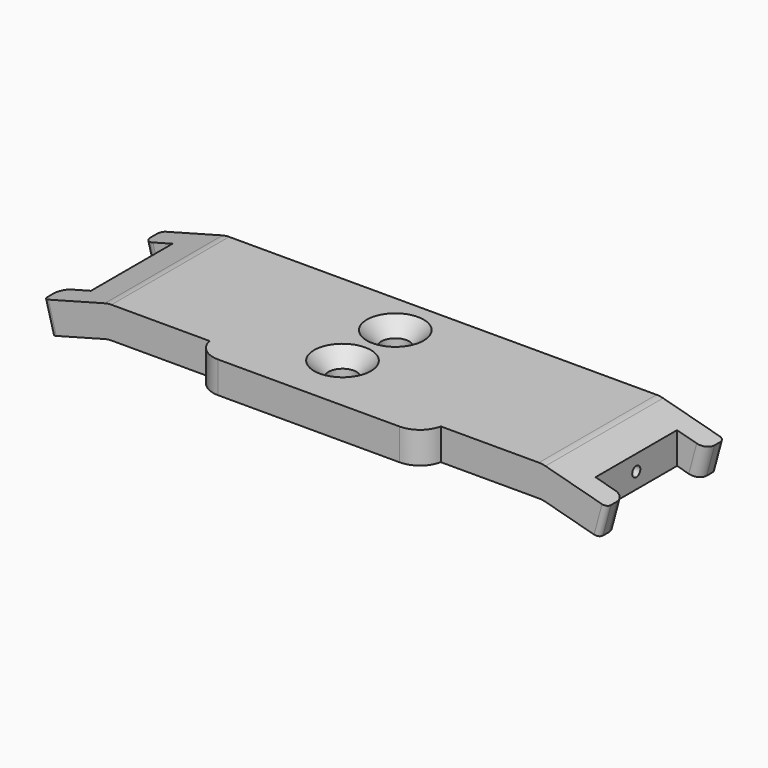
from build123d import *

# Parameters (mm, degrees)
F1_DEPTH        = 29
F2_W            = 45.6076951546
F2_H            = 6.2116570825
F3_DEPTH        = 4
F4_W            = 14.4515829202
F4_H            = 20.1
F4_W_2          = 11.8
F5_DEPTH        = 25
F7_D            = 2
F7_DEPTH        = 5
F7_TIP          = 0.600860619
F8_T1_DEPTH     = 29
F8_T3_DEPTH     = 29
F8_T5_DEPTH     = 32.2913124397
F8_T7_DEPTH     = 32.2913124397
F8_T9_DEPTH     = 30.7065545103
F8_T11_DEPTH    = 30.7065545103
F9_R            = 1
F11_D           = 2
F11_DEPTH       = 5
F11_TIP         = 0.600860619
F12_R           = 2
F14_D           = 5.5
F14_CSINK_D     = 11.2
F14_CSINK_ANGLE = 90


# Not quite as in the source:
# - a fillet or chamfer that OpenCascade refuses, or shapes differently, is made with other operations: its cross-section is extruded or revolved along the edge and cut away or added


with BuildPart() as f1:
    # F0 (on Front) → F1 (new body)
    with BuildSketch(Plane.XZ):
        Polygon((45.541646846, 20.7590438725), (-40.0660483086, 20.7590438725), (-52.8151150019, 17.3429417477), (-51.2622007313, 11.54738679), (-40.0660483086, 14.54738679), (45.541646846, 14.54738679), (56.7377992687, 11.54738679), (58.2907135393, 17.3429417477), align=None)
    extrude(amount=F1_DEPTH)

    # F2 (on face) → F3 (join)
    with BuildSketch(Plane.XZ.offset(29)):
        with Locations((2.7377992687, 17.6532153312)):
            Rectangle(F2_W, F2_H)
    extrude(amount=F3_DEPTH)

    # F4 (on face) → F5 (cut)
    with BuildSketch(Plane.XY.offset(20.7590438725)):
        with Locations((-54.240906462, -14.5)):
            Rectangle(F4_W, F4_H)
        with Locations((58.3907135393, -14.5)):
            Rectangle(F4_W_2, F4_H)
    extrude(amount=-F5_DEPTH, mode=Mode.SUBTRACT)

    # F7
    with Locations(Plane(origin=(-47.0151150019, 0, 0), x_dir=(0, -1, 0), z_dir=(-1, 0, 0))):
        with Locations((14.5, 15.7970470638)):
            Hole(F7_D / 2, depth=F7_DEPTH)
            with Locations((0, 0, -(F7_DEPTH + F7_TIP / 2))):  # 118° drill point
                Cone(0, F7_D / 2, F7_TIP, mode=Mode.SUBTRACT)

    # F8: fillet of radius 5 on 6 edges, made by hand

    # F8_s2 → F8_t1 (join)
    with BuildSketch(Plane.XZ):
        with BuildLine():
            ThreePointArc((46.1774795836, 14.3770159214), (45.5360153192, 14.5046110969), (44.8833843581, 14.54738679))
            Line((44.8833843581, 14.54738679), (45.541646846, 14.54738679))
            Line((45.541646846, 14.54738679), (46.1774795836, 14.3770159214))
        make_face()
    extrude(amount=F8_T1_DEPTH)

    # F8_s4 → F8_t3 (join)
    with BuildSketch(Plane.XZ):
        with BuildLine():
            ThreePointArc((-39.4077858206, 14.54738679), (-40.0604167817, 14.5046110969), (-40.7018810462, 14.3770159214))
            Line((-40.7018810462, 14.3770159214), (-40.0660483086, 14.54738679))
            Line((-40.0660483086, 14.54738679), (-39.4077858206, 14.54738679))
        make_face()
    extrude(amount=F8_T3_DEPTH)

    # F8_s6 → F8_t5 (cut)
    with BuildSketch(Plane.XZ.offset(-1.6456562198)):
        with BuildLine():
            ThreePointArc((44.8833843581, 20.7590438725), (45.5360153192, 20.7162681793), (46.1774795836, 20.5886730039))
            Line((46.1774795836, 20.5886730039), (45.541646846, 20.7590438725))
            Line((45.541646846, 20.7590438725), (44.8833843581, 20.7590438725))
        make_face()
    extrude(amount=F8_T5_DEPTH, mode=Mode.SUBTRACT)

    # F8_s8 → F8_t7 (cut)
    with BuildSketch(Plane.XZ.offset(-1.6456562198)):
        with BuildLine():
            ThreePointArc((-39.4077858206, 20.7590438725), (-40.0604167817, 20.7162681793), (-40.7018810462, 20.5886730039))
            Line((-40.7018810462, 20.5886730039), (-40.0660483086, 20.7590438725))
            Line((-40.0660483086, 20.7590438725), (-39.4077858206, 20.7590438725))
        make_face()
    extrude(amount=F8_T7_DEPTH, mode=Mode.SUBTRACT)

    # F8_s10 → F8_t9 (cut)
    with BuildSketch(Plane.XY.offset(2.2999380761)):
        with BuildLine():
            ThreePointArc((20.6426673604, -33), (23.8049450206, -31.8729833462), (25.541646846, -29))
            Line((25.541646846, -29), (25.541646846, -33))
            Line((25.541646846, -33), (20.6426673604, -33))
        make_face()
    extrude(amount=F8_T9_DEPTH, mode=Mode.SUBTRACT)

    # F8_s12 → F8_t11 (cut)
    with BuildSketch(Plane.XY.offset(2.2999380761)):
        with BuildLine():
            ThreePointArc((-20.0660483086, -29), (-18.3293464832, -31.8729833462), (-15.167068823, -33))
            Line((-15.167068823, -33), (-20.0660483086, -33))
            Line((-20.0660483086, -33), (-20.0660483086, -29))
        make_face()
    extrude(amount=F8_T11_DEPTH, mode=Mode.SUBTRACT)

    # F9
    f9_edges = [f1.edges().sort_by_distance(p)[0] for p in [
        (-52.038658, -29, 14.445164),
        (-52.038658, 0, 14.445164),
        (57.514256, 0, 14.445164),
        (57.514256, -29, 14.445164),
    ]]
    fillet(f9_edges, radius=F9_R)

    # F11
    with Locations(Plane.YZ.offset(52.4907135393)):
        with Locations((-14.5, 15.7970470638)):
            Hole(F11_D / 2, depth=F11_DEPTH)
            with Locations((0, 0, -(F11_DEPTH + F11_TIP / 2))):  # 118° drill point
                Cone(0, F11_D / 2, F11_TIP, mode=Mode.SUBTRACT)

    # F12
    f12_edges = [f1.edges().sort_by_distance(p)[0] for p in [
        (-52.038658, -24.55, 14.445164),
        (-52.038658, -4.45, 14.445164),
        (57.514256, -24.55, 14.445164),
        (57.514256, -4.45, 14.445164),
    ]]
    fillet(f12_edges, radius=F12_R)

    # F14 (through all)
    with Locations(Plane.XY.offset(20.7590438725)):
        with Locations((0, -21.3), (0, -8.3)):
            CounterSinkHole(F14_D / 2, F14_CSINK_D / 2, counter_sink_angle=F14_CSINK_ANGLE)


solid = f1.part
